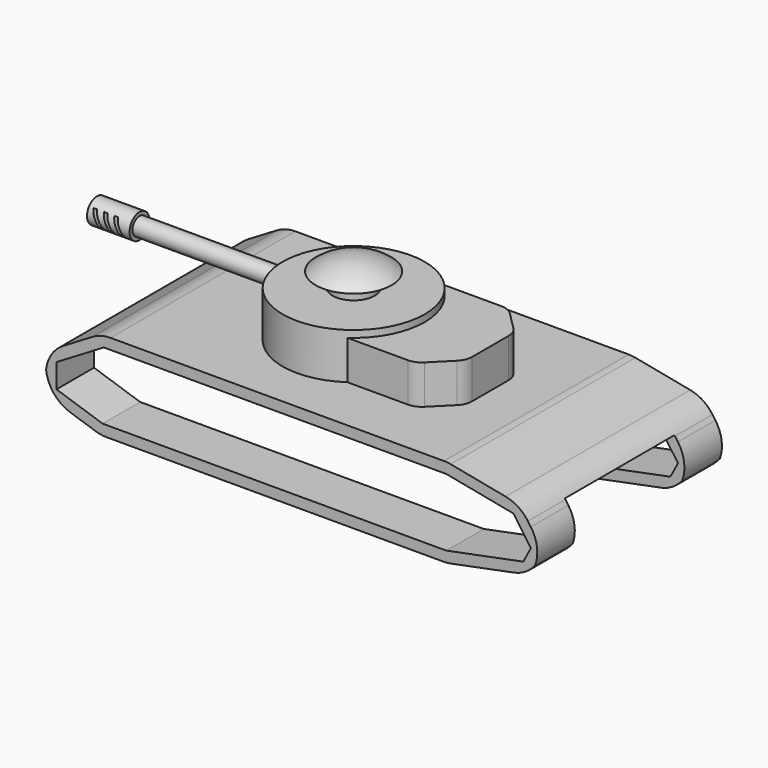
from build123d import *

# Parameters (mm, degrees)
F1_DEPTH      = 32.5
F0_W          = 5.9106643312
F0_H          = 4.1622407734
F5_R          = 2.5
F6_DEPTH      = 65.3
F8_R          = 3.5
F8_R_2        = 1.9092401518
F9_DEPTH      = 12
F12_DEPTH     = 12.5
F13_DEPTH     = 59.6
F14_T1_DEPTH  = 78.7900561948
F14_T3_DEPTH  = 93.3821225166
F14_T5_DEPTH  = 101.1499908241
F14_T7_DEPTH  = 73.0383114632
F14_T9_DEPTH  = 69.9303599295
F14_T11_DEPTH = 88.6692573472
F14_T13_DEPTH = 95.8474480124
F14_T15_DEPTH = 85.0967001073
F14_T17_DEPTH = 69.7853101798
F16_DEPTH     = 65.001
F17_W         = 38.5783538222
F17_H         = 35.981696099
F18_DEPTH     = 80
F21_DEPTH     = 13.5
F22_SIZE      = 8
F23_R         = 5


# Not quite as in the source:
# - a fillet or chamfer that OpenCascade refuses, or shapes differently, is made with other operations: its cross-section is extruded or revolved along the edge and cut away or added


with BuildPart() as f1:
    # F0 (on Front) → F1 (new body, symmetric)
    with BuildSketch(Plane.XZ):
        Polygon((-45.1924055815, 0), (0, 0), (52.3890219629, 0), (75.743816793, 4.6511264518), (79.4435888529, 11.5881953388), (72.7377533913, 21.0688542575), (52.3890219629, 24.9998606741), (20.0160350651, 24.9998606741), (0, 24.9998606741), (-20.0160350651, 24.9998606741), (-45.1924055815, 24.9998606741), (-60.6851913035, 15.7504361123), (-60.6851913035, 5.1135984249), align=None)
    extrude(amount=F1_DEPTH, both=True)

    # F0 (on Front) → F2 (revolve)
    with BuildSketch(Plane.XZ):
        Polygon((0, 24.9998606741), (20.0160350651, 24.9998606741), (20.0160350651, 37.9490554333), (5.9106643312, 37.9490554333), (5.9106643312, 33.7868146598), (0, 33.7868146598), align=None)
        with Locations((2.9553321656, 35.8679350466)):
            Rectangle(F0_W, F0_H)
    revolve(axis=Axis((0, 0, 31.4744580537), (0, 0, -1)))

    # F0 (on Front) → F3 (revolve)
    with BuildSketch(Plane.XZ):
        with Locations((2.9553321656, 40.03017582)):
            Rectangle(F0_W, F0_H)
    revolve(axis=Axis((0, 0, 40.03017582), (0, 0, -1)))

    # F0 (on Front) → F4 (revolve)
    with BuildSketch(Plane.XZ):
        with BuildLine():
            Line((0, 42.1112962067), (5.9106643312, 42.1112962067))
            Line((5.9106643312, 42.1112962067), (10.6915488715, 42.1112962067))
            ThreePointArc((10.6915488715, 42.1112962067), (5.6799749875, 44.9003117854), (0, 45.6955254889))
            Line((0, 45.6955254889), (0, 42.1112962067))
        make_face()
    revolve(axis=Axis((0, 0, 44.0255403519), (0, 0, 1)))

    # F5 (on Right) → F6 (join)
    with BuildSketch(Plane.YZ):
        with Locations((0, 33.6981996664)):
            Circle(F5_R)
    extrude(amount=-F6_DEPTH)

    # F8 (on offset) → F9 (join)
    with BuildSketch(Plane(origin=(-72.3, 0, 0), x_dir=(0, -1, 0), z_dir=(-1, 0, 0))):
        with Locations((0, 33.6981996664)):
            Circle(F8_R)
        with Locations((0, 33.6981996664)):
            Circle(F8_R_2, mode=Mode.SUBTRACT)
    extrude(amount=-F9_DEPTH)

    # F11 (on face) → F12 (cut, symmetric)
    with BuildSketch(Plane.XZ):
        Polygon((-68.1971950683, 31.44), (-70.0017480406, 35.8125706637), (-71.008284801, 35.8125706637), (-69.2037318287, 31.44), align=None)
        Polygon((-65.27, 31.44), (-67.0745529723, 35.8125706637), (-68.0810897328, 35.8125706637), (-66.2765367604, 31.44), align=None)
        Polygon((-62.3428049317, 31.44), (-64.1473579041, 35.8125706637), (-65.1538946645, 35.8125706637), (-63.3493416922, 31.44), align=None)
    extrude(amount=F12_DEPTH, both=True, mode=Mode.SUBTRACT)

    # F8 (on offset) → F13 (cut)
    with BuildSketch(Plane(origin=(-72.3, 0, 0), x_dir=(0, -1, 0), z_dir=(-1, 0, 0))):
        with Locations((0, 33.6981996664)):
            Circle(F8_R_2)
    extrude(amount=-F13_DEPTH, mode=Mode.SUBTRACT)

    # F14: fillet of radius 10 on 9 edges, made by hand

    # F14_s2 → F14_t1 (cut)
    with BuildSketch(Plane.XZ.offset(-39.3950280974)):
        with BuildLine():
            ThreePointArc((-42.4343943425, 24.9998606741), (-45.0931383524, 24.6399374524), (-47.5604936203, 23.5860767321))
            Line((-47.5604936203, 23.5860767321), (-45.1924055815, 24.9998606741))
            Line((-45.1924055815, 24.9998606741), (-42.4343943425, 24.9998606741))
        make_face()
    extrude(amount=F14_T1_DEPTH, mode=Mode.SUBTRACT)

    # F14_s4 → F14_t3 (cut)
    with BuildSketch(Plane.XZ.offset(-46.6910612583)):
        with BuildLine():
            ThreePointArc((-60.6851913035, 10.074011609), (-59.3817708834, 15.0105593512), (-55.8112905813, 18.660227667))
            Line((-55.8112905813, 18.660227667), (-60.6851913035, 15.7504361123))
            Line((-60.6851913035, 15.7504361123), (-60.6851913035, 10.074011609))
        make_face()
    extrude(amount=F14_T3_DEPTH, mode=Mode.SUBTRACT)

    # F14_s6 → F14_t5 (cut)
    with BuildSketch(Plane.XZ.offset(-50.5749954121)):
        with BuildLine():
            ThreePointArc((-53.819507052, 2.847488714), (-58.788991569, 6.484550485), (-60.6851913035, 12.3435965898))
            Line((-60.6851913035, 12.3435965898), (-60.6851913035, 5.1135984249))
            Line((-60.6851913035, 5.1135984249), (-53.819507052, 2.847488714))
        make_face()
    extrude(amount=F14_T5_DEPTH, mode=Mode.SUBTRACT)

    # F14_s8 → F14_t7 (cut)
    with BuildSketch(Plane.XZ.offset(-36.5191557316)):
        with BuildLine():
            ThreePointArc((-43.5847432888, 0), (-45.172024178, 0.126776647), (-46.7190590373, 0.5038921242))
            Line((-46.7190590373, 0.5038921242), (-45.1924055815, 0))
            Line((-45.1924055815, 0), (-43.5847432888, 0))
        make_face()
    extrude(amount=F14_T7_DEPTH, mode=Mode.SUBTRACT)

    # F14_s10 → F14_t9 (cut)
    with BuildSketch(Plane.XZ.offset(-34.9651799647)):
        with BuildLine():
            ThreePointArc((53.3561027034, 0.1925949188), (52.3842626661, 0.0482652062), (51.402949977, 0))
            Line((51.402949977, 0), (52.3890219629, 0))
            Line((52.3890219629, 0), (53.3561027034, 0.1925949188))
        make_face()
    extrude(amount=F14_T9_DEPTH, mode=Mode.SUBTRACT)

    # F14_s12 → F14_t11 (cut)
    with BuildSketch(Plane.XZ.offset(-44.3346286736)):
        with BuildLine():
            ThreePointArc((77.9715125335, 8.8280537222), (75.1095772753, 5.505276407), (71.1011368974, 3.7265329614))
            Line((71.1011368974, 3.7265329614), (75.743816793, 4.6511264518))
            Line((75.743816793, 4.6511264518), (77.9715125335, 8.8280537222))
        make_face()
    extrude(amount=F14_T11_DEPTH, mode=Mode.SUBTRACT)

    # F14_s14 → F14_t13 (cut)
    with BuildSketch(Plane.XZ.offset(-47.9237240062)):
        with BuildLine():
            ThreePointArc((75.8809250083, 16.6250622505), (77.6970376868, 11.4783126325), (76.5402984143, 6.1445286899))
            Line((76.5402984143, 6.1445286899), (79.4435888529, 11.5881953388))
            Line((79.4435888529, 11.5881953388), (75.8809250083, 16.6250622505))
        make_face()
    extrude(amount=F14_T13_DEPTH, mode=Mode.SUBTRACT)

    # F14_s16 → F14_t15 (cut)
    with BuildSketch(Plane.XZ.offset(-42.5483500536)):
        with BuildLine():
            ThreePointArc((68.7913767646, 21.8312227568), (72.3162104373, 20.4155165159), (75.0587812714, 17.7874027817))
            Line((75.0587812714, 17.7874027817), (72.7377533913, 21.0688542575))
            Line((72.7377533913, 21.0688542575), (68.7913767646, 21.8312227568))
        make_face()
    extrude(amount=F14_T15_DEPTH, mode=Mode.SUBTRACT)

    # F14_s18 → F14_t17 (cut)
    with BuildSketch(Plane.XZ.offset(-34.8926550899)):
        with BuildLine():
            ThreePointArc((51.4319599269, 24.9998606741), (52.3846686566, 24.9543745285), (53.3287103766, 24.8183298894))
            Line((53.3287103766, 24.8183298894), (52.3890219629, 24.9998606741))
            Line((52.3890219629, 24.9998606741), (51.4319599269, 24.9998606741))
        make_face()
    extrude(amount=F14_T17_DEPTH, mode=Mode.SUBTRACT)

    # F15 (on face) → F16 (cut, through all)
    with BuildSketch(Plane(origin=(0, 32.5, 0), x_dir=(-1, 0, 0), z_dir=(0, 1, 0))):
        Polygon((-75.9255432126, 11.3668606403), (-73.7650670064, 7.315969929), (-52.0932003671, 3), (0, 3), (44.7101068937, 3), (57.6851913035, 7.2825978744), (57.6851913035, 14.0475087613), (44.3650022098, 21.9998606741), (0, 21.9998606741), (-52.1019033521, 21.9998606741), (-70.9848152684, 18.3520240427), align=None)
    extrude(amount=-F16_DEPTH, mode=Mode.SUBTRACT)

    # F17 (on Right) → F18 (cut, symmetric)
    with BuildSketch(Plane.YZ):
        Rectangle(F17_W, F17_H)
    extrude(amount=F18_DEPTH, both=True, mode=Mode.SUBTRACT)

    # F20 (on offset) → F21 (join, symmetric)
    with BuildSketch(Plane.YZ.offset(25)):
        Polygon((-16.4748225361, 24.9998606741), (0, 24.9998606741), (16.4748225361, 24.9998606741), (16.4748225361, 36.0052287579), (0, 36.0052287579), (-16.4748225361, 36.0052287579), align=None)
    extrude(amount=F21_DEPTH, both=True)

    # F22
    f22_edges = [f1.edges().sort_by_distance(p)[0] for p in [
        (38.5, 16.474823, 30.502545),
        (38.5, -16.474823, 30.502545),
    ]]
    chamfer(f22_edges, length=F22_SIZE)

    # F23
    f23_edges = [f1.edges().sort_by_distance(p)[0] for p in [
        (38.5, -8.474823, 30.502545),
        (30.5, -16.474823, 30.502545),
        (38.5, 8.474823, 30.502545),
        (30.5, 16.474823, 30.502545),
    ]]
    fillet(f23_edges, radius=F23_R)


solid = f1.part
